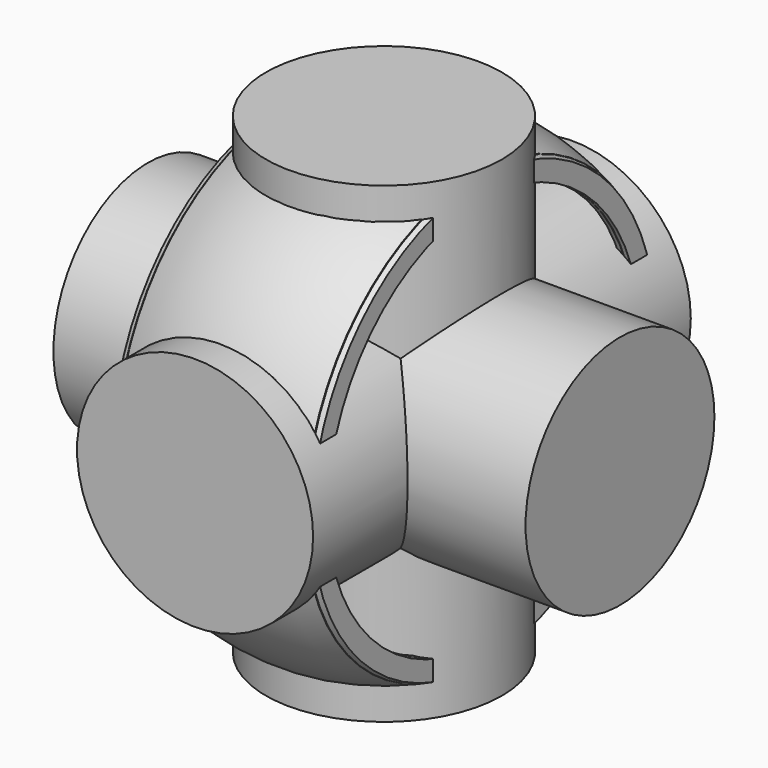
from build123d import *

# Parameters (mm, degrees)
F2_R     = 125
F5_DEPTH = 250
F3_R     = 125
F6_DEPTH = 250
F1_R     = 125
F7_DEPTH = 250


with BuildPart() as f4:
    # F0 (on Top) → F4 (revolve)
    with BuildSketch(Plane.XY):
        with BuildLine():
            Line((-100.5, 206.1547847478), (-100.5, 228.9099167795))
            ThreePointArc((-100.5, 228.9099167795), (-103.0062036193, 227.7931562096), (-105.5, 226.6489576415))
            Line((-105.5, 226.6489576415), (-105.5, 215.5684346095))
            Line((-105.5, 215.5684346095), (-105.5, 206.1547847478))
            Line((-105.5, 206.1547847478), (-100.5, 206.1547847478))
        make_face()
    revolve(axis=Axis((0, 0, 0), (1, 0, 0)))


with BuildPart() as f4b:
    # F0 (on Top) → F4, piece 2 (revolve)
    with BuildSketch(Plane.XY):
        with BuildLine():
            Line((-95, 225), (-95, 225.8317958127))
            ThreePointArc((-95, 225.8317958127), (-90.0216753203, 227.8620152033), (-85, 229.7825058615))
            ThreePointArc((-85, 229.7825058615), (-67.3162801965, 235.5706229998), (-49.244289009, 240))
            ThreePointArc((-49.244289009, 240), (-29.7190418638, 243.1908274395), (-10, 244.7958332979))
            Line((-10, 244.7958332979), (-10, 245))
            Line((-10, 245), (3.458e-07, 245))
            Line((3.458e-07, 245), (10, 245))
            Line((10, 245), (10, 244.7958332979))
            ThreePointArc((10, 244.7958332979), (29.7190418638, 243.1908274395), (49.244289009, 240))
            ThreePointArc((49.244289009, 240), (67.3162801965, 235.5706229998), (85, 229.7825058615))
            ThreePointArc((85, 229.7825058615), (90.0216753203, 227.8620152033), (95, 225.8317958127))
            Line((95, 225.8317958127), (95, 225))
            Line((95, 225), (95, 206.1547847478))
            Line((95, 206.1547847478), (100, 206.1547847478))
            Line((100, 206.1547847478), (100, 229.1287847478))
            ThreePointArc((100, 229.1287847478), (0, 250), (-100, 229.1287847478))
            Line((-100, 229.1287847478), (-100, 206.1547847478))
            Line((-100, 206.1547847478), (-95, 206.1547847478))
            Line((-95, 206.1547847478), (-95, 225))
        make_face()
    revolve(axis=Axis((0, 0, 0), (1, 0, 0)))


with BuildPart() as f4c:
    # F0 (on Top) → F4, piece 3 (revolve)
    with BuildSketch(Plane.XY):
        with BuildLine():
            ThreePointArc((105.5, 226.6489576415), (103.0062036193, 227.7931562096), (100.5, 228.9099167795))
            Line((100.5, 228.9099167795), (100.5, 206.1547847478))
            Line((100.5, 206.1547847478), (105.5, 206.1547847478))
            Line((105.5, 206.1547847478), (105.5, 215.5684346095))
            Line((105.5, 215.5684346095), (105.5, 226.6489576415))
        make_face()
    revolve(axis=Axis((0, 0, 0), (1, 0, 0)))


with BuildPart() as f5:
    # F2 (on Front) → F5 (new body, symmetric)
    with BuildSketch(Plane.XZ):
        Circle(F2_R)
    extrude(amount=F5_DEPTH, both=True)

    # F3 (on Top) → F6 (join, symmetric)
    with BuildSketch(Plane.XY):
        Circle(F3_R)
    extrude(amount=F6_DEPTH, both=True)

    # F1 (on Right) → F7 (join, symmetric)
    with BuildSketch(Plane.YZ):
        Circle(F1_R)
    extrude(amount=F7_DEPTH, both=True)


solid = Compound([f4.part, f4b.part, f4c.part, f5.part])
